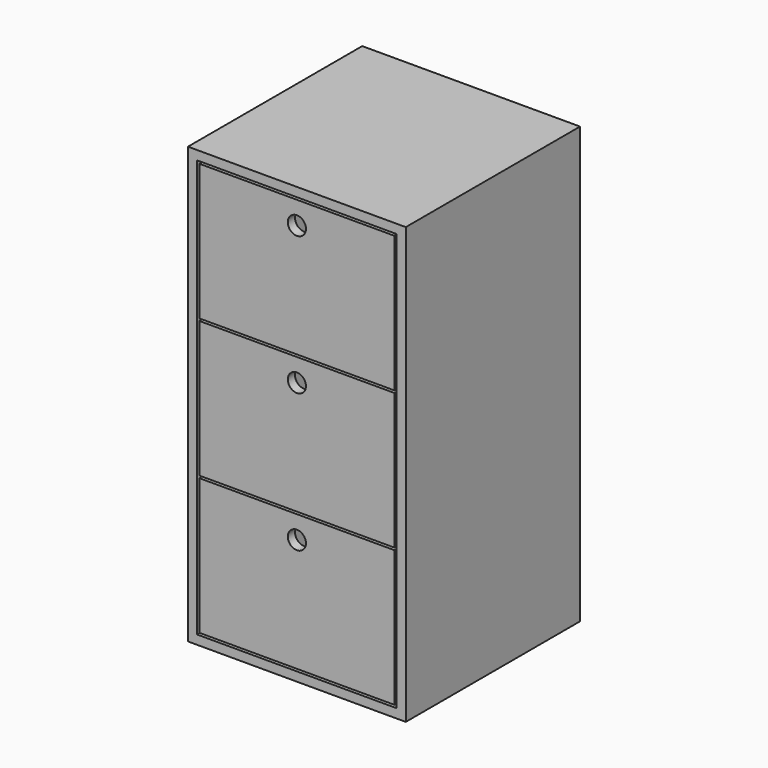
from build123d import *

# Parameters (mm, degrees)
F3_W     = 304.8
F3_H     = 304.8
F4_DEPTH = 609.6
F5_W     = 279.4
F5_H     = 584.2
F6_DEPTH = 292.1
F8_W     = 273.05
F8_H     = 190.5
F8_R     = 12.7
F9_DEPTH = 12.7


# Not quite as in the source:
# - a length typed as a fraction of an inch, garbled in the dataset ("3 / 203.2 mm" for 3/8 in), is restored
# - a feature names something its author has since deleted; it is built from what else it names


with BuildPart() as f4:
    # F3 (on Top) → F4 (new body)
    with BuildSketch(Plane.XY):
        Rectangle(F3_W, F3_H)
    extrude(amount=F4_DEPTH)

    # F5 (on face) → F6 (cut)
    with BuildSketch(Plane.XZ.offset(152.4)):
        with Locations((0, 304.8)):
            Rectangle(F5_W, F5_H)
    extrude(amount=-F6_DEPTH, mode=Mode.SUBTRACT)


with BuildPart() as f9:
    # F8 (on offset) → F9 (new body)
    with BuildSketch(Plane.XZ.offset(152.4)):
        with Locations((0, 498.475)):
            Rectangle(F8_W, F8_H)
        with Locations((0, 561.975)):
            Circle(F8_R, mode=Mode.SUBTRACT)
    extrude(amount=-F9_DEPTH)


with BuildPart() as f9b:
    # F8 (on offset) → F9, piece 2 (new body)
    with BuildSketch(Plane.XZ.offset(152.4)):
        with Locations((0, 304.8)):
            Rectangle(F8_W, F8_H)
        with Locations((0, 368.3)):
            Circle(F8_R, mode=Mode.SUBTRACT)
    extrude(amount=-F9_DEPTH)


with BuildPart() as f9c:
    # F8 (on offset) → F9, piece 3 (new body)
    with BuildSketch(Plane.XZ.offset(152.4)):
        with Locations((0, 111.125)):
            Rectangle(F8_W, F8_H)
        with Locations((0, 174.625)):
            Circle(F8_R, mode=Mode.SUBTRACT)
    extrude(amount=-F9_DEPTH)


solid = Compound([f4.part, f9.part, f9b.part, f9c.part])
